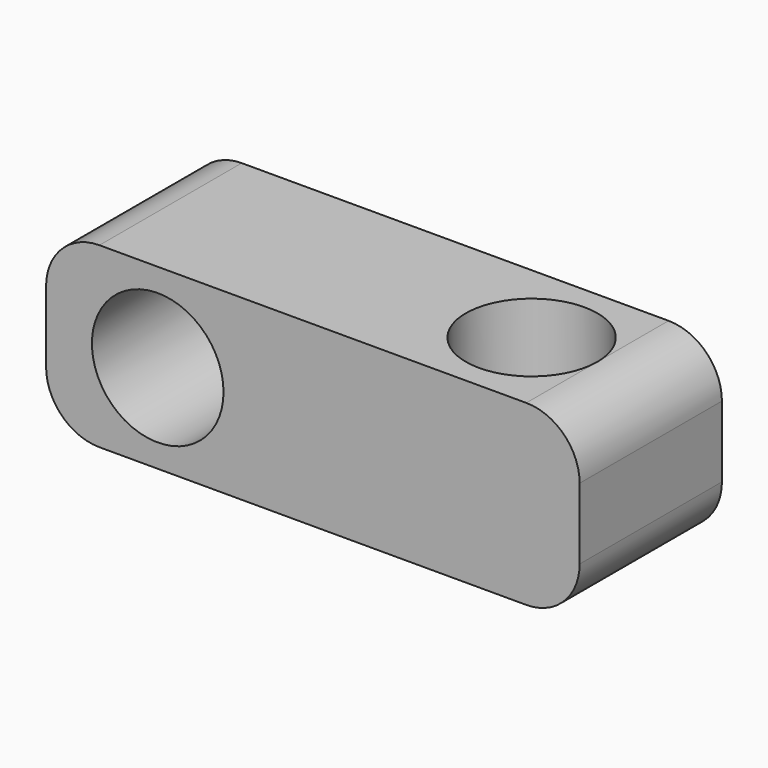
from build123d import *

# Parameters (mm, degrees)
F0_W     = 30
F0_H     = 10
F1_DEPTH = 10
F2_R     = 3.7
F3_DEPTH = 10
F4_R     = 3.7
F5_DEPTH = 10
F6_R     = 2.99999


# Not quite as in the source:
# - a fillet or chamfer is up to 0.001 mm smaller than in the source, because OpenCascade refuses the exact size


with BuildPart() as f1:
    # F0 (on Top) → F1 (new body)
    with BuildSketch(Plane.XY):
        Rectangle(F0_W, F0_H)
    extrude(amount=F1_DEPTH)

    # F2 (on face) → F3 (cut, through all)
    with BuildSketch(Plane.XY.offset(10)):
        with Locations((8.3, 0)):
            Circle(F2_R)
    extrude(amount=-F3_DEPTH, mode=Mode.SUBTRACT)

    # F4 (on face) → F5 (cut, through all)
    with BuildSketch(Plane.XZ.offset(5)):
        with Locations((-8.7227521392, 5)):
            Circle(F4_R)
    extrude(amount=-F5_DEPTH, mode=Mode.SUBTRACT)

    # F6 (radius 3 in the source; OpenCascade refuses exactly that, so slightly less here)
    f6_edges = [f1.edges().sort_by_distance(p)[0] for p in [
        (-15, 0, 10),
        (15, 0, 10),
        (15, 0, 0),
        (-15, 0, 0),
    ]]
    fillet(f6_edges, radius=F6_R)


solid = f1.part
